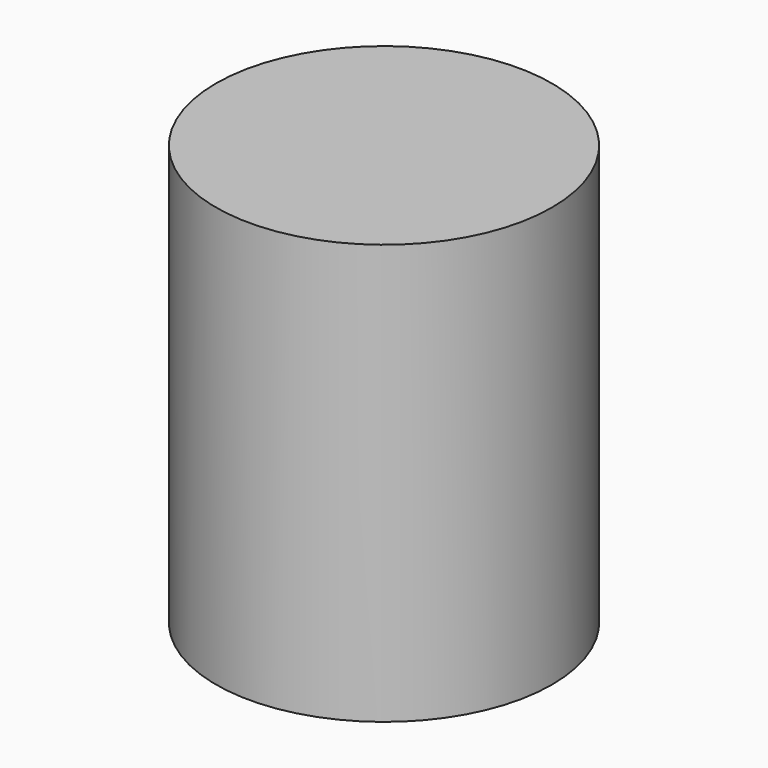
from build123d import *

# Parameters (mm, degrees)
F0_R     = 300
F1_DEPTH = 750


# Not quite as in the source:
# - the program builds the solid bodies; features that only make, move or delete a surface that nothing else refers to are left out


with BuildPart() as f1:
    # F0 (on Top) → F1 (new body)
    with BuildSketch(Plane.XY):
        Circle(F0_R)
    extrude(amount=F1_DEPTH)


solid = f1.part
